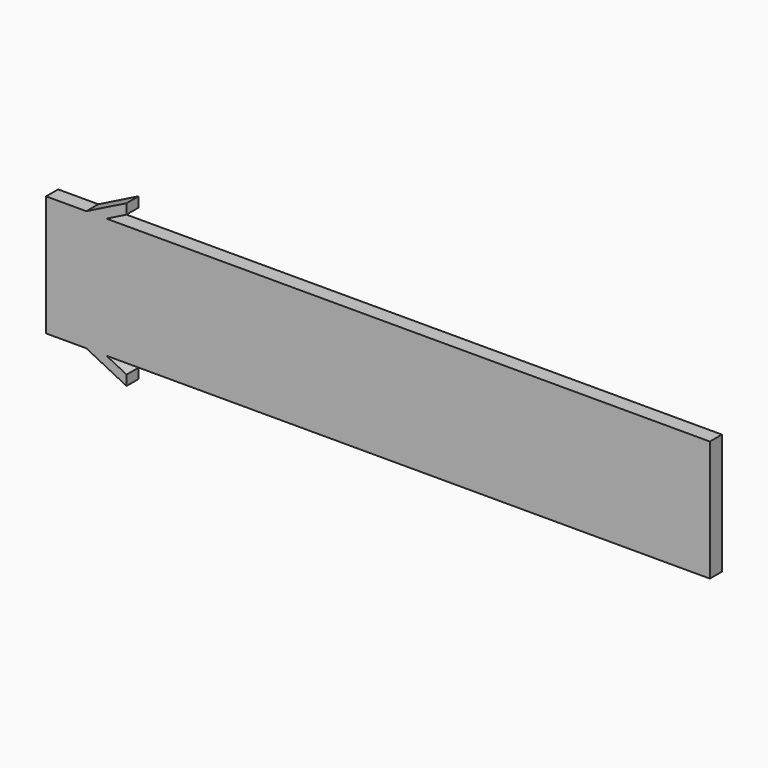
from build123d import *

# Parameters (mm, degrees)
F0_W      = 0.75
F0_H      = 6
F1_DEPTH  = 33
F2_R      = 1
F3_DEPTH  = 2
F4_R      = 1
F5_W      = 2
F5_H      = 0.75
F6_DEPTH  = 1
F7_SIZE2  = 1.99999
F7_SIZE   = 0.99999
F8_W      = 2
F8_H      = 0.75
F9_DEPTH  = 1
F10_SIZE2 = 1.99999
F10_SIZE  = 0.99999
F12_DEPTH = 25


# Not quite as in the source:
# - a fillet or chamfer is up to 0.001 mm smaller than in the source, because OpenCascade refuses the exact size


with BuildPart() as f1:
    # F0 (on Right) → F1 (new body)
    with BuildSketch(Plane.YZ):
        with Locations((-8.76496256, 0.0332817435)):
            Rectangle(F0_W, F0_H)
    extrude(amount=F1_DEPTH)

    # F2 (on face) → F3 (join)
    with BuildSketch(Plane(origin=(0, -8.38996256, 0), x_dir=(-1, 0, 0), z_dir=(0, 1, 0))):
        with Locations((-9, 0.0332817435)):
            Circle(F2_R)
        with Locations((-24, 0.0332817435)):
            Circle(F2_R)
    extrude(amount=F3_DEPTH)

    # F4
    f4_edges = [f1.edges().sort_by_distance(p)[0] for p in [
        (10, -6.389963, 0.033282),
        (25, -6.389963, 0.033282),
    ]]
    fillet(f4_edges, radius=F4_R)

    # F5 (on face) → F6 (join)
    with BuildSketch(Plane.XY.offset(3.0332817435)):
        with Locations((3, -8.76496256)):
            Rectangle(F5_W, F5_H)
    extrude(amount=F6_DEPTH)

    # F7 (size 1 and 2 in the source; OpenCascade refuses exactly that, so slightly less here)
    f7_edges = [f1.edges().sort_by_distance(p)[0] for p in [
        (2, -8.764963, 4.033282),
    ]]
    f7_side = f1.faces().sort_by_distance((2, -8.764963, 3.533282))[0]
    chamfer(f7_edges, length=F7_SIZE, length2=F7_SIZE2, reference=f7_side)

    # F8 (on face) → F9 (join)
    with BuildSketch(Plane(origin=(0, 0, -2.9667182565), x_dir=(1, 0, 0), z_dir=(0, 0, -1))):
        with Locations((3, 8.76496256)):
            Rectangle(F8_W, F8_H)
    extrude(amount=F9_DEPTH)

    # F10 (size 1 and 2 in the source; OpenCascade refuses exactly that, so slightly less here)
    f10_edges = [f1.edges().sort_by_distance(p)[0] for p in [
        (2, -8.764963, -3.966718),
    ]]
    f10_side = f1.faces().sort_by_distance((2, -8.764963, -3.466718))[0]
    chamfer(f10_edges, length=F10_SIZE, length2=F10_SIZE2, reference=f10_side)

    # F11 (on face) → F12 (cut)
    with BuildSketch(Plane(origin=(0, -8.38996256, 0), x_dir=(-1, 0, 0), z_dir=(0, 1, 0))):
        Polygon((-3, 3.0332817435), (-4, 3.5332817435), (-4, 3.0332817435), align=None)
        Polygon((-3, -2.9667182565), (-4, -2.9667182565), (-4, -3.4667182565), align=None)
    extrude(amount=-F12_DEPTH, mode=Mode.SUBTRACT)


solid = f1.part
